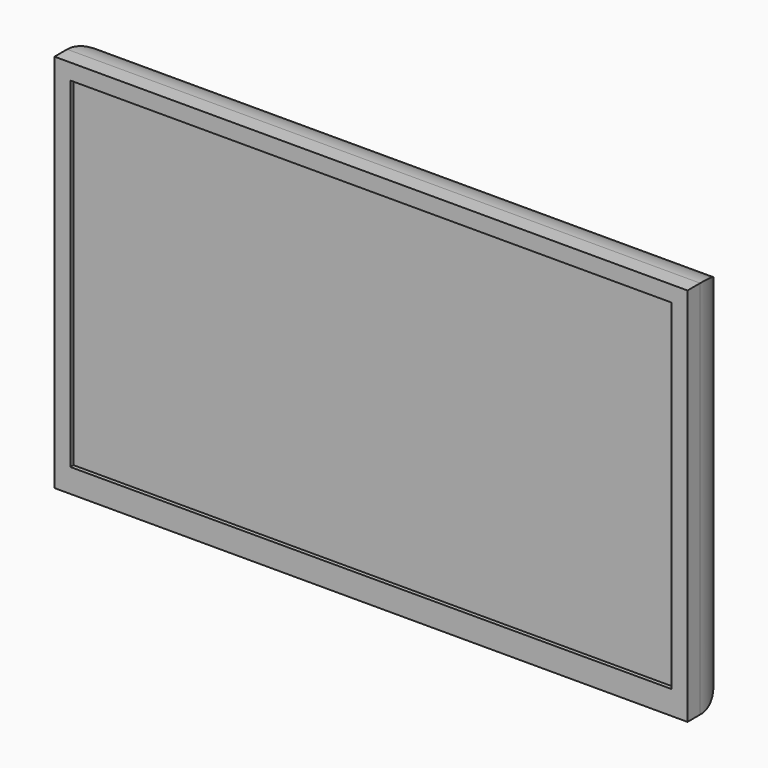
from build123d import *

# Parameters (mm, degrees)
F0_W        = 508
F0_H        = 304.8
F1_DEPTH    = 50.8
F2_W        = 482.6
F2_H        = 273.05
F3_DEPTH    = 3.175
F4_R        = 2
F5_DEPTH    = 15
F6_W        = 88.9
F6_H        = 22.225
F7_DEPTH    = 25.4
F8_T1_DEPTH = 400.05
F8_T3_DEPTH = 495.3
F8_T5_DEPTH = 698.5
F8_T7_DEPTH = 400.05


# Not quite as in the source:
# - a fillet or chamfer that OpenCascade refuses, or shapes differently, is made with other operations: its cross-section is extruded or revolved along the edge and cut away or added


with BuildPart() as f1:
    # F0 (on Front) → F1 (new body)
    with BuildSketch(Plane.XZ):
        with Locations((0, 152.4)):
            Rectangle(F0_W, F0_H)
    extrude(amount=F1_DEPTH)

    # F2 (on face) → F3 (cut)
    with BuildSketch(Plane.XZ.offset(50.8)):
        with Locations((0, 155.575)):
            Rectangle(F2_W, F2_H)
    extrude(amount=-F3_DEPTH, mode=Mode.SUBTRACT)

    # F4 (on face) → F5 (cut)
    with BuildSketch(Plane(origin=(0, 0, 0), x_dir=(-1, 0, 0), z_dir=(0, 1, 0))):
        with Locations((-50, 207.95)):
            Circle(F4_R)
        with Locations((50, 207.95)):
            Circle(F4_R)
        with Locations((-50, 107.95)):
            Circle(F4_R)
        with Locations((50, 107.95)):
            Circle(F4_R)
    extrude(amount=-F5_DEPTH, mode=Mode.SUBTRACT)

    # F6 (on face) → F7 (cut)
    with BuildSketch(Plane(origin=(0, 0, 0), x_dir=(-1, 0, 0), z_dir=(0, 1, 0))):
        Polygon((177.8, 98.425), (-177.8, 98.425), (-177.8, 22.225), (-44.45, 22.225), (44.45, 22.225), (177.8, 22.225), align=None)
        with Locations((0, 11.1125)):
            Rectangle(F6_W, F6_H)
    extrude(amount=-F7_DEPTH, mode=Mode.SUBTRACT)

    # F8: fillet of radius 38.1 on 5 edges, made by hand

    # F8_s2 → F8_t1 (cut)
    with BuildSketch(Plane.YZ.offset(-50.8)):
        with BuildLine():
            ThreePointArc((-38.1, 0), (-11.1592316368, 11.1592316368), (0, 38.1))
            Line((0, 38.1), (0, 0))
            Line((0, 0), (-38.1, 0))
        make_face()
    extrude(amount=F8_T1_DEPTH, mode=Mode.SUBTRACT)

    # F8_s4 → F8_t3 (cut)
    with BuildSketch(Plane.XY.offset(-95.25)):
        with BuildLine():
            ThreePointArc((215.9, 0), (242.8407683632, -11.1592316368), (254, -38.1))
            Line((254, -38.1), (254, 0))
            Line((254, 0), (215.9, 0))
        make_face()
        with BuildLine():
            ThreePointArc((-254, -38.1), (-242.8407683632, -11.1592316368), (-215.9, 0))
            Line((-215.9, 0), (-254, 0))
            Line((-254, 0), (-254, -38.1))
        make_face()
    extrude(amount=F8_T3_DEPTH, mode=Mode.SUBTRACT)

    # F8_s6 → F8_t5 (cut)
    with BuildSketch(Plane.YZ.offset(-349.25)):
        with BuildLine():
            ThreePointArc((-38.1, 304.8), (-11.1592316368, 293.6407683632), (0, 266.7))
            Line((0, 266.7), (0, 304.8))
            Line((0, 304.8), (-38.1, 304.8))
        make_face()
    extrude(amount=F8_T5_DEPTH, mode=Mode.SUBTRACT)

    # F8_s8 → F8_t7 (cut)
    with BuildSketch(Plane.YZ.offset(-349.25)):
        with BuildLine():
            ThreePointArc((-38.1, 0), (-11.1592316368, 11.1592316368), (0, 38.1))
            Line((0, 38.1), (0, 0))
            Line((0, 0), (-38.1, 0))
        make_face()
    extrude(amount=F8_T7_DEPTH, mode=Mode.SUBTRACT)


solid = f1.part
